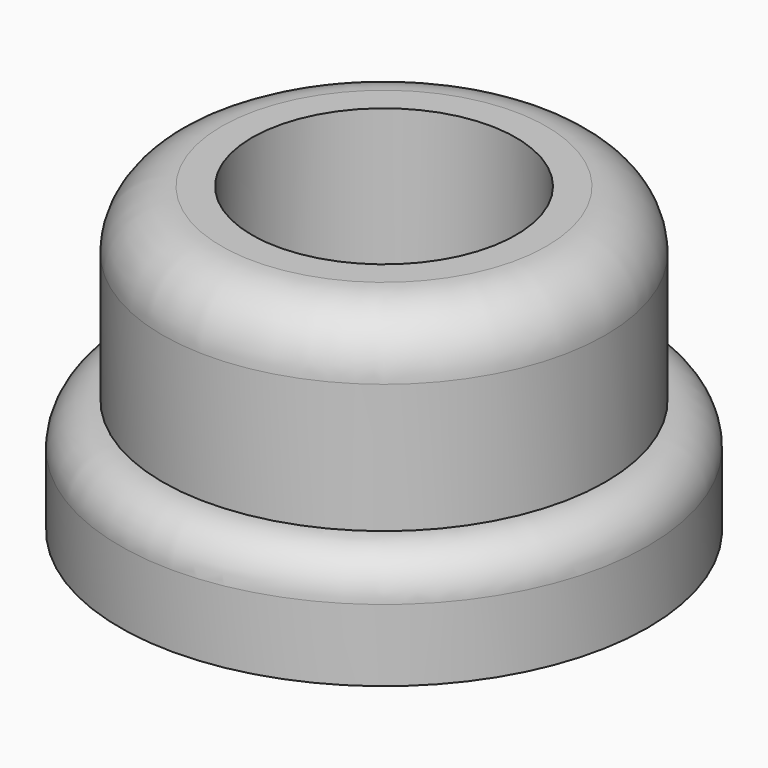
from build123d import *

# Parameters (mm, degrees)
F0_R     = 15
F1_DEPTH = 6.5
F2_R     = 2.4142135624
F4_D     = 15
F5_T     = -0.7
F7_DEPTH = 10.6984395534
F8_R     = 3.3542973282


with BuildPart() as f1:
    # F0 (on Top) → F1 (new body)
    with BuildSketch(Plane.XY):
        Circle(F0_R)
    extrude(amount=F1_DEPTH)

    # F2
    f2_edges = [f1.edges().sort_by_distance(p)[0] for p in [
        (-15, 0, 6.5),
    ]]
    fillet(f2_edges, radius=F2_R)

    # F4 (through all)
    with Locations(Plane(origin=(0, 0, 0), x_dir=(1, 0, 0), z_dir=(0, 0, -1))):
        with Locations((0, 0)):
            Hole(F4_D / 2)

    # F5
    f5_openings = [f1.faces().sort_by_distance(p)[0] for p in [
        (-14.575736, 0, 0),
    ]]
    offset(amount=F5_T, openings=f5_openings)

    # F7 (add): a face of the model
    f7_faces = [f1.faces().sort_by_distance(p)[0] for p in [
        (-12.2298066402, 0, 6.5),
    ]]
    extrude(f7_faces, amount=F7_DEPTH)

    # F8
    f8_edges = [f1.edges().sort_by_distance(p)[0] for p in [
        (-12.585786, 0, 17.19844),
    ]]
    fillet(f8_edges, radius=F8_R)


solid = f1.part
